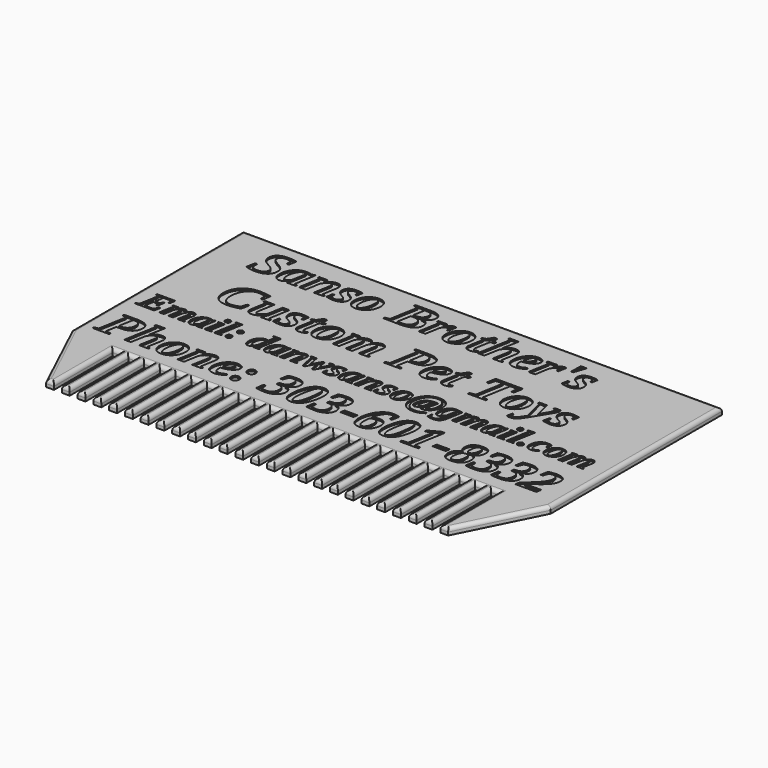
from build123d import *

# Parameters (mm, degrees)
F1_DEPTH       = 1.2
F2_R           = 0.65
F3_TEXT_SIZE   = 8.9951780656
F3_TEXT_SIZE_2 = 6.2498474158
F3_TEXT_SIZE_3 = 8.932777361
F4_DEPTH       = 0.3


# Not quite as in the source:
# - Text() gives the source's letters only with a copy of the font that has no kerning and outlines rounded to 1/6400 em; it was checked with that copy


with BuildPart() as f1:
    # F0 (on Top) → F1 (new body)
    with BuildSketch(Plane.XY):
        Polygon((59, -42.5), (-26, -42.5), (-26, -80.5), (-19.4, -94.5), (-18, -94.5), (-18, -81.5), (-16.6, -81.5), (-16.6, -94.5), (-15.2, -94.5), (-15.2, -81.5), (-13.8, -81.5), (-13.8, -94.5), (-12.4, -94.5), (-12.4, -81.5), (-11, -81.5), (-11, -94.5), (-9.6, -94.5), (-9.6, -81.5), (-8.2, -81.5), (-8.2, -94.5), (-6.8, -94.5), (-6.8, -81.5), (-5.4, -81.5), (-5.4, -94.5), (-4, -94.5), (-4, -81.5), (-2.6, -81.5), (-2.6, -94.5), (-1.2, -94.5), (-1.2, -81.5), (0.2, -81.5), (0.2, -94.5), (1.6, -94.5), (1.6, -81.5), (3, -81.5), (3, -94.5), (4.4, -94.5), (4.4, -81.5), (5.8, -81.5), (5.8, -94.5), (7.2, -94.5), (7.2, -81.5), (8.6, -81.5), (8.6, -94.5), (10, -94.5), (10, -81.5), (11.4, -81.5), (11.4, -94.5), (12.8, -94.5), (12.8, -81.5), (14.2, -81.5), (14.2, -94.5), (15.6, -94.5), (15.6, -81.5), (17, -81.5), (17, -94.5), (18.4, -94.5), (18.4, -81.5), (19.8, -81.5), (19.8, -94.5), (21.2, -94.5), (21.2, -81.5), (22.6, -81.5), (22.6, -94.5), (24, -94.5), (24, -81.5), (25.4, -81.5), (25.4, -94.5), (26.8, -94.5), (26.8, -81.5), (28.2, -81.5), (28.2, -94.5), (29.6, -94.5), (29.6, -81.5), (31, -81.5), (31, -94.5), (32.4, -94.5), (32.4, -81.5), (33.8, -81.5), (33.8, -94.5), (35.2, -94.5), (35.2, -81.5), (36.6, -81.5), (36.6, -94.5), (38, -94.5), (38, -81.5), (39.4, -81.5), (39.4, -94.5), (40.8, -94.5), (40.8, -81.5), (42.2, -81.5), (42.2, -94.5), (43.6, -94.5), (43.6, -81.5), (45, -81.5), (45, -94.5), (46.4, -94.5), (46.4, -81.5), (47.8, -81.5), (47.8, -94.5), (49.2, -94.5), (49.2, -81.5), (50.6, -81.5), (50.6, -94.5), (52, -94.5), (59, -80.5), align=None)
    extrude(amount=F1_DEPTH)

    # F2
    f2_edges = [f1.edges().sort_by_distance(p)[0] for p in [
        (-15.9, -94.5, 1.2),
        (16.5, -42.5, 1.2),
        (-26, -61.5, 1.2),
        (-22.7, -87.5, 1.2),
        (-18.7, -94.5, 1.2),
        (-18, -88, 1.2),
        (-17.3, -81.5, 1.2),
        (-16.6, -88, 1.2),
        (-15.2, -88, 1.2),
        (-14.5, -81.5, 1.2),
        (-13.8, -88, 1.2),
        (-13.1, -94.5, 1.2),
        (-12.4, -88, 1.2),
        (-11.7, -81.5, 1.2),
        (-11, -88, 1.2),
        (-10.3, -94.5, 1.2),
        (-9.6, -88, 1.2),
        (-8.9, -81.5, 1.2),
        (-8.2, -88, 1.2),
        (-7.5, -94.5, 1.2),
        (-6.8, -88, 1.2),
        (-6.1, -81.5, 1.2),
        (-5.4, -88, 1.2),
        (-4.7, -94.5, 1.2),
        (-4, -88, 1.2),
        (-3.3, -81.5, 1.2),
        (-2.6, -88, 1.2),
        (-1.9, -94.5, 1.2),
        (-1.2, -88, 1.2),
        (-0.5, -81.5, 1.2),
        (0.2, -88, 1.2),
        (0.9, -94.5, 1.2),
        (1.6, -88, 1.2),
        (2.3, -81.5, 1.2),
        (3, -88, 1.2),
        (3.7, -94.5, 1.2),
        (4.4, -88, 1.2),
        (5.1, -81.5, 1.2),
        (5.8, -88, 1.2),
        (6.5, -94.5, 1.2),
        (7.2, -88, 1.2),
        (7.9, -81.5, 1.2),
        (8.6, -88, 1.2),
        (9.3, -94.5, 1.2),
        (10, -88, 1.2),
        (10.7, -81.5, 1.2),
        (11.4, -88, 1.2),
        (12.1, -94.5, 1.2),
        (12.8, -88, 1.2),
        (13.5, -81.5, 1.2),
        (14.2, -88, 1.2),
        (14.9, -94.5, 1.2),
        (15.6, -88, 1.2),
        (16.3, -81.5, 1.2),
        (17, -88, 1.2),
        (17.7, -94.5, 1.2),
        (18.4, -88, 1.2),
        (19.1, -81.5, 1.2),
        (19.8, -88, 1.2),
        (20.5, -94.5, 1.2),
        (21.2, -88, 1.2),
        (21.9, -81.5, 1.2),
        (22.6, -88, 1.2),
        (23.3, -94.5, 1.2),
        (24, -88, 1.2),
        (24.7, -81.5, 1.2),
        (25.4, -88, 1.2),
        (26.1, -94.5, 1.2),
        (26.8, -88, 1.2),
        (27.5, -81.5, 1.2),
        (28.2, -88, 1.2),
        (28.9, -94.5, 1.2),
        (29.6, -88, 1.2),
        (30.3, -81.5, 1.2),
        (31, -88, 1.2),
        (31.7, -94.5, 1.2),
        (32.4, -88, 1.2),
        (33.1, -81.5, 1.2),
        (33.8, -88, 1.2),
        (34.5, -94.5, 1.2),
        (35.2, -88, 1.2),
        (35.9, -81.5, 1.2),
        (36.6, -88, 1.2),
        (37.3, -94.5, 1.2),
        (38, -88, 1.2),
        (38.7, -81.5, 1.2),
        (39.4, -88, 1.2),
        (40.1, -94.5, 1.2),
        (40.8, -88, 1.2),
        (41.5, -81.5, 1.2),
        (42.2, -88, 1.2),
        (42.9, -94.5, 1.2),
        (43.6, -88, 1.2),
        (44.3, -81.5, 1.2),
        (45, -88, 1.2),
        (45.7, -94.5, 1.2),
        (46.4, -88, 1.2),
        (47.1, -81.5, 1.2),
        (47.8, -88, 1.2),
        (48.5, -94.5, 1.2),
        (49.2, -88, 1.2),
        (49.9, -81.5, 1.2),
        (50.6, -88, 1.2),
        (51.3, -94.5, 1.2),
        (55.5, -87.5, 1.2),
        (59, -61.5, 1.2),
    ]]
    fillet(f2_edges, radius=F2_R)

    # F3 (on face) → F4 (cut)
    with BuildSketch(Plane.XY.offset(1.2)):
        with Locations((-19, -50.9765282072)):
            Text("Sanso Brother's", F3_TEXT_SIZE, font='Tinos', font_style=FontStyle.BOLDITALIC, text_align=(TextAlign.LEFT, TextAlign.BOTTOM))
        with Locations((-16.7512054836, -61.3209829827)):
            Text('Custom Pet Toys', F3_TEXT_SIZE, font='Tinos', font_style=FontStyle.BOLDITALIC, text_align=(TextAlign.LEFT, TextAlign.BOTTOM))
        with Locations((-24, -68.9998901394)):
            Text('Email: danwsanso@gmail.com', F3_TEXT_SIZE_2, font='Tinos', font_style=FontStyle.BOLDITALIC, text_align=(TextAlign.LEFT, TextAlign.BOTTOM))
        with Locations((-24, -78.4315996999)):
            Text('Phone: 303-601-8332', F3_TEXT_SIZE_3, font='Tinos', font_style=FontStyle.BOLDITALIC, text_align=(TextAlign.LEFT, TextAlign.BOTTOM))
    extrude(amount=-F4_DEPTH, mode=Mode.SUBTRACT)


solid = f1.part
